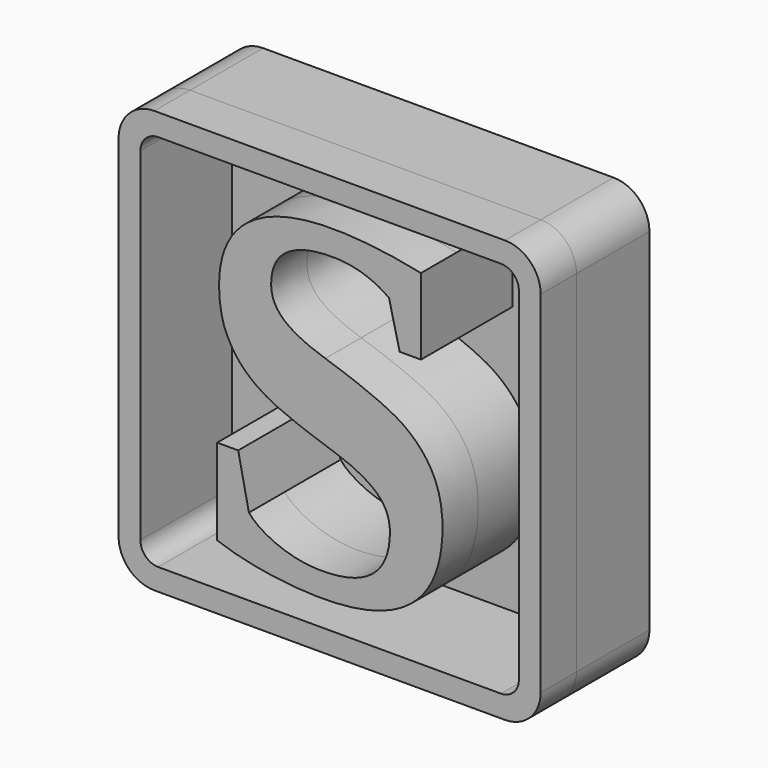
from build123d import *

# Parameters (mm, degrees)
F0_TEXT_SIZE = 69.4972222222
F1_DEPTH     = 9.906
F2_W         = 59.944
F2_H         = 59.944
F3_DEPTH     = 3.048
F4_W         = 59.944
F4_H         = 59.944
F4_W_2       = 53.7464
F4_H_2       = 53.7464
F5_DEPTH     = 9.906
F6_R         = 5.08
F7_R         = 2.54
F8_DEPTH     = 6.35


# Not quite as in the source:
# - Text() gives the source's letters only with a copy of the font that has no kerning and outlines rounded to 1/6400 em; it was checked with that copy


with BuildPart() as f1:
    # F0 (on Front) → F1 (new body)
    with BuildSketch(Plane.XZ):
        with Locations((-36.3391012755, -18.474436296)):
            Text('S', F0_TEXT_SIZE, font='Tinos', font_style=FontStyle.BOLD, text_align=(TextAlign.LEFT, TextAlign.BOTTOM))
    extrude(amount=F1_DEPTH)

    # F2 (on face) → F3 (join)
    with BuildSketch(Plane(origin=(0, 0, 0), x_dir=(-1, 0, 0), z_dir=(0, 1, 0))):
        with Locations((16.6670807534, 4.0664761014)):
            Rectangle(F2_W, F2_H)
        with BuildLine():
            Line((29.6499936366, -4.5315560877), (32.6362024039, -4.5315560877))
            Line((32.6362024039, -4.5315560877), (32.6362024039, -16.7478646815))
            add(Edge.make_bspline(
                [(25.6701917703, -18.496154178), (29.7260062234, -17.8337587787), (32.6362024039, -16.7478646815)],
                knots=[0, 0, 0, 1, 1, 1], degree=2))
            add(Edge.make_bspline(
                [(17.7051585671, -19.1585495773), (21.6143773171, -19.1585495773), (25.6701917703, -18.496154178)],
                knots=[0, 0, 0, 1, 1, 1], degree=2))
            add(Edge.make_bspline(
                [(0.6349033588, -4.6618633794), (0.6349033588, -19.1585495773), (17.7051585671, -19.1585495773)],
                knots=[0, 0, 0, 1, 1, 1], degree=2))
            add(Edge.make_bspline(
                [(2.1660140359, 1.8860780269), (0.6349033588, -0.893810862), (0.6349033588, -4.6618633794)],
                knots=[0, 0, 0, 1, 1, 1], degree=2))
            add(Edge.make_bspline(
                [(6.5964619525, 6.5499931744), (3.697124713, 4.6659669158), (2.1660140359, 1.8860780269)],
                knots=[0, 0, 0, 1, 1, 1], degree=2))
            add(Edge.make_bspline(
                [(17.2708009282, 10.9858705616), (9.4957991921, 8.4340194331), (6.5964619525, 6.5499931744)],
                knots=[0, 0, 0, 1, 1, 1], degree=2))
            add(Edge.make_bspline(
                [(23.1020522303, 13.8472015078), (21.2343143831, 12.2346487734), (17.2708009282, 10.9858705616)],
                knots=[0, 0, 0, 1, 1, 1], degree=2))
            add(Edge.make_bspline(
                [(24.9697900775, 17.7292729053), (24.9697900775, 15.4597542422), (23.1020522303, 13.8472015078)],
                knots=[0, 0, 0, 1, 1, 1], degree=2))
            add(Edge.make_bspline(
                [(22.7328482373, 22.4692006397), (24.9697900775, 20.9218015512), (24.9697900775, 17.7292729053)],
                knots=[0, 0, 0, 1, 1, 1], degree=2))
            add(Edge.make_bspline(
                [(16.3152141227, 24.0165997283), (20.495906397, 24.0165997283), (22.7328482373, 22.4692006397)],
                knots=[0, 0, 0, 1, 1, 1], degree=2))
            add(Edge.make_bspline(
                [(8.2361620394, 21.4973254227), (11.7001642095, 24.0165997283), (16.3152141227, 24.0165997283)],
                knots=[0, 0, 0, 1, 1, 1], degree=2))
            Line((8.2361620394, 21.4973254227), (6.7159103032, 15.2534343637))
            Line((6.7159103032, 15.2534343637), (3.697124713, 15.2534343637))
            Line((3.697124713, 15.2534343637), (3.697124713, 26.079798513))
            add(Edge.make_bspline(
                [(16.3152141227, 27.5457555442), (10.6142701123, 27.5457555442), (3.697124713, 26.079798513)],
                knots=[0, 0, 0, 1, 1, 1], degree=2))
            add(Edge.make_bspline(
                [(28.2763376036, 24.4020921328), (24.1879463275, 27.5457555442), (16.3152141227, 27.5457555442)],
                knots=[0, 0, 0, 1, 1, 1], degree=2))
            add(Edge.make_bspline(
                [(32.3647288796, 15.2534343637), (32.3647288796, 21.2584287213), (28.2763376036, 24.4020921328)],
                knots=[0, 0, 0, 1, 1, 1], degree=2))
            add(Edge.make_bspline(
                [(31.3168410758, 9.5416314123), (32.3647288796, 11.8654447803), (32.3647288796, 15.2534343637)],
                knots=[0, 0, 0, 1, 1, 1], degree=2))
            add(Edge.make_bspline(
                [(28.504375364, 5.5889768984), (30.268953272, 7.2178180442), (31.3168410758, 9.5416314123)],
                knots=[0, 0, 0, 1, 1, 1], degree=2))
            add(Edge.make_bspline(
                [(24.1770873866, 2.7547933047), (26.739797456, 3.9601357526), (28.504375364, 5.5889768984)],
                knots=[0, 0, 0, 1, 1, 1], degree=2))
            add(Edge.make_bspline(
                [(15.7722670741, -0.3834406363), (21.6143773171, 1.5494508567), (24.1770873866, 2.7547933047)],
                knots=[0, 0, 0, 1, 1, 1], degree=2))
            add(Edge.make_bspline(
                [(9.9573041835, -3.4728093429), (11.8087536192, -1.7408082578), (15.7722670741, -0.3834406363)],
                knots=[0, 0, 0, 1, 1, 1], degree=2))
            add(Edge.make_bspline(
                [(8.1058547477, -7.7132257926), (8.1058547477, -5.204810428), (9.9573041835, -3.4728093429)],
                knots=[0, 0, 0, 1, 1, 1], degree=2))
            add(Edge.make_bspline(
                [(17.8463247998, -15.7271242301), (8.1058547477, -15.7271242301), (8.1058547477, -7.7132257926)],
                knots=[0, 0, 0, 1, 1, 1], degree=2))
            add(Edge.make_bspline(
                [(23.813312864, -14.6086533099), (20.9302640359, -15.7271242301), (17.8463247998, -15.7271242301)],
                knots=[0, 0, 0, 1, 1, 1], degree=2))
            add(Edge.make_bspline(
                [(28.1297419005, -11.8179054801), (26.6963616921, -13.4901823898), (23.813312864, -14.6086533099)],
                knots=[0, 0, 0, 1, 1, 1], degree=2))
            Line((28.1297419005, -11.8179054801), (29.6499936366, -4.5315560877))
        make_face(mode=Mode.SUBTRACT)
        with BuildLine():
            Line((32.6362024039, -16.7478646815), (32.6362024039, -4.5315560877))
            Line((32.6362024039, -4.5315560877), (29.6499936366, -4.5315560877))
            Line((29.6499936366, -4.5315560877), (28.1297419005, -11.8179054801))
            add(Edge.make_bspline(
                [(28.1297419005, -11.8179054801), (26.6963616921, -13.4901823898), (23.813312864, -14.6086533099)],
                knots=[0, 0, 0, 1, 1, 1], degree=2))
            add(Edge.make_bspline(
                [(23.813312864, -14.6086533099), (20.9302640359, -15.7271242301), (17.8463247998, -15.7271242301)],
                knots=[0, 0, 0, 1, 1, 1], degree=2))
            add(Edge.make_bspline(
                [(17.8463247998, -15.7271242301), (8.1058547477, -15.7271242301), (8.1058547477, -7.7132257926)],
                knots=[0, 0, 0, 1, 1, 1], degree=2))
            add(Edge.make_bspline(
                [(8.1058547477, -7.7132257926), (8.1058547477, -5.204810428), (9.9573041835, -3.4728093429)],
                knots=[0, 0, 0, 1, 1, 1], degree=2))
            add(Edge.make_bspline(
                [(9.9573041835, -3.4728093429), (11.8087536192, -1.7408082578), (15.7722670741, -0.3834406363)],
                knots=[0, 0, 0, 1, 1, 1], degree=2))
            add(Edge.make_bspline(
                [(15.7722670741, -0.3834406363), (21.6143773171, 1.5494508567), (24.1770873866, 2.7547933047)],
                knots=[0, 0, 0, 1, 1, 1], degree=2))
            add(Edge.make_bspline(
                [(24.1770873866, 2.7547933047), (26.739797456, 3.9601357526), (28.504375364, 5.5889768984)],
                knots=[0, 0, 0, 1, 1, 1], degree=2))
            add(Edge.make_bspline(
                [(28.504375364, 5.5889768984), (30.268953272, 7.2178180442), (31.3168410758, 9.5416314123)],
                knots=[0, 0, 0, 1, 1, 1], degree=2))
            add(Edge.make_bspline(
                [(31.3168410758, 9.5416314123), (32.3647288796, 11.8654447803), (32.3647288796, 15.2534343637)],
                knots=[0, 0, 0, 1, 1, 1], degree=2))
            add(Edge.make_bspline(
                [(32.3647288796, 15.2534343637), (32.3647288796, 21.2584287213), (28.2763376036, 24.4020921328)],
                knots=[0, 0, 0, 1, 1, 1], degree=2))
            add(Edge.make_bspline(
                [(28.2763376036, 24.4020921328), (24.1879463275, 27.5457555442), (16.3152141227, 27.5457555442)],
                knots=[0, 0, 0, 1, 1, 1], degree=2))
            add(Edge.make_bspline(
                [(16.3152141227, 27.5457555442), (10.6142701123, 27.5457555442), (3.697124713, 26.079798513)],
                knots=[0, 0, 0, 1, 1, 1], degree=2))
            Line((3.697124713, 26.079798513), (3.697124713, 15.2534343637))
            Line((3.697124713, 15.2534343637), (6.7159103032, 15.2534343637))
            Line((6.7159103032, 15.2534343637), (8.2361620394, 21.4973254227))
            add(Edge.make_bspline(
                [(8.2361620394, 21.4973254227), (11.7001642095, 24.0165997283), (16.3152141227, 24.0165997283)],
                knots=[0, 0, 0, 1, 1, 1], degree=2))
            add(Edge.make_bspline(
                [(16.3152141227, 24.0165997283), (20.495906397, 24.0165997283), (22.7328482373, 22.4692006397)],
                knots=[0, 0, 0, 1, 1, 1], degree=2))
            add(Edge.make_bspline(
                [(22.7328482373, 22.4692006397), (24.9697900775, 20.9218015512), (24.9697900775, 17.7292729053)],
                knots=[0, 0, 0, 1, 1, 1], degree=2))
            add(Edge.make_bspline(
                [(24.9697900775, 17.7292729053), (24.9697900775, 15.4597542422), (23.1020522303, 13.8472015078)],
                knots=[0, 0, 0, 1, 1, 1], degree=2))
            add(Edge.make_bspline(
                [(23.1020522303, 13.8472015078), (21.2343143831, 12.2346487734), (17.2708009282, 10.9858705616)],
                knots=[0, 0, 0, 1, 1, 1], degree=2))
            add(Edge.make_bspline(
                [(17.2708009282, 10.9858705616), (9.4957991921, 8.4340194331), (6.5964619525, 6.5499931744)],
                knots=[0, 0, 0, 1, 1, 1], degree=2))
            add(Edge.make_bspline(
                [(6.5964619525, 6.5499931744), (3.697124713, 4.6659669158), (2.1660140359, 1.8860780269)],
                knots=[0, 0, 0, 1, 1, 1], degree=2))
            add(Edge.make_bspline(
                [(2.1660140359, 1.8860780269), (0.6349033588, -0.893810862), (0.6349033588, -4.6618633794)],
                knots=[0, 0, 0, 1, 1, 1], degree=2))
            add(Edge.make_bspline(
                [(0.6349033588, -4.6618633794), (0.6349033588, -19.1585495773), (17.7051585671, -19.1585495773)],
                knots=[0, 0, 0, 1, 1, 1], degree=2))
            add(Edge.make_bspline(
                [(17.7051585671, -19.1585495773), (21.6143773171, -19.1585495773), (25.6701917703, -18.496154178)],
                knots=[0, 0, 0, 1, 1, 1], degree=2))
            add(Edge.make_bspline(
                [(25.6701917703, -18.496154178), (29.7260062234, -17.8337587787), (32.6362024039, -16.7478646815)],
                knots=[0, 0, 0, 1, 1, 1], degree=2))
        make_face()
    extrude(amount=F3_DEPTH)

    # F4 (on face) → F5 (join)
    with BuildSketch(Plane.XZ):
        with Locations((-16.6670807534, 4.0664761014)):
            Rectangle(F4_W, F4_H)
        with Locations((-16.6670807534, 4.0664761014)):
            Rectangle(F4_W_2, F4_H_2, mode=Mode.SUBTRACT)
    extrude(amount=F5_DEPTH)

    # F6
    f6_edges = [f1.edges().sort_by_distance(p)[0] for p in [
        (13.304919, -3.429, 34.038476),
        (-46.639081, -3.429, 34.038476),
        (-46.639081, -3.429, -25.905524),
        (13.304919, -3.429, -25.905524),
    ]]
    fillet(f6_edges, radius=F6_R)

    # F7
    f7_edges = [f1.edges().sort_by_distance(p)[0] for p in [
        (-43.540281, -4.953, 30.939676),
        (10.206119, -4.953, 30.939676),
        (10.206119, -4.953, -22.806724),
        (-43.540281, -4.953, -22.806724),
    ]]
    fillet(f7_edges, radius=F7_R)

    # F8 (add): faces of the model
    f8_faces = [f1.faces().sort_by_distance(p)[0] for p in [
        (-16.8746488624, -9.906, 4.1006522746),
        (11.0538554244, -9.906, 4.0664761014),
    ]]
    extrude(f8_faces, amount=F8_DEPTH)


solid = f1.part
